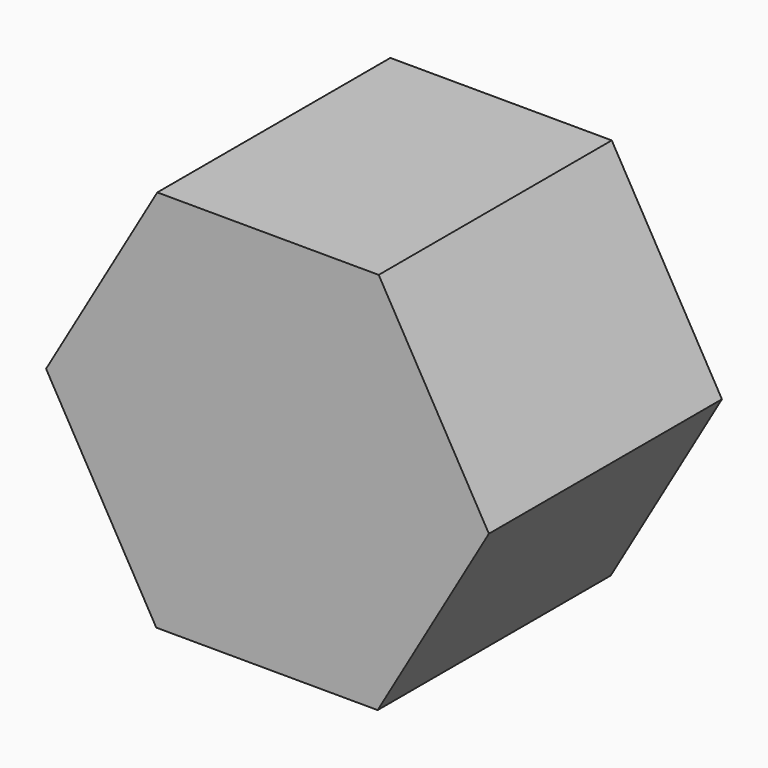
from build123d import *

# Parameters (mm, degrees)
F2_DEPTH = 4.7752


# Not quite as in the source:
# - a variable given as a bare number and used for a length is read in inches; the dataset says mm whatever the document's units were


with BuildPart() as f2:
    # F1 (on Front) → F2 (new body)
    with BuildSketch(Plane.XZ):
        Polygon((3.6294990207, -0.0098797008), (1.8233055822, 3.1382985046), (-1.8061934385, 3.1481782053), (-3.6294990207, 0.0098797008), (-1.8233055822, -3.1382985046), (1.8061934385, -3.1481782053), align=None)
    extrude(amount=F2_DEPTH)


solid = f2.part
